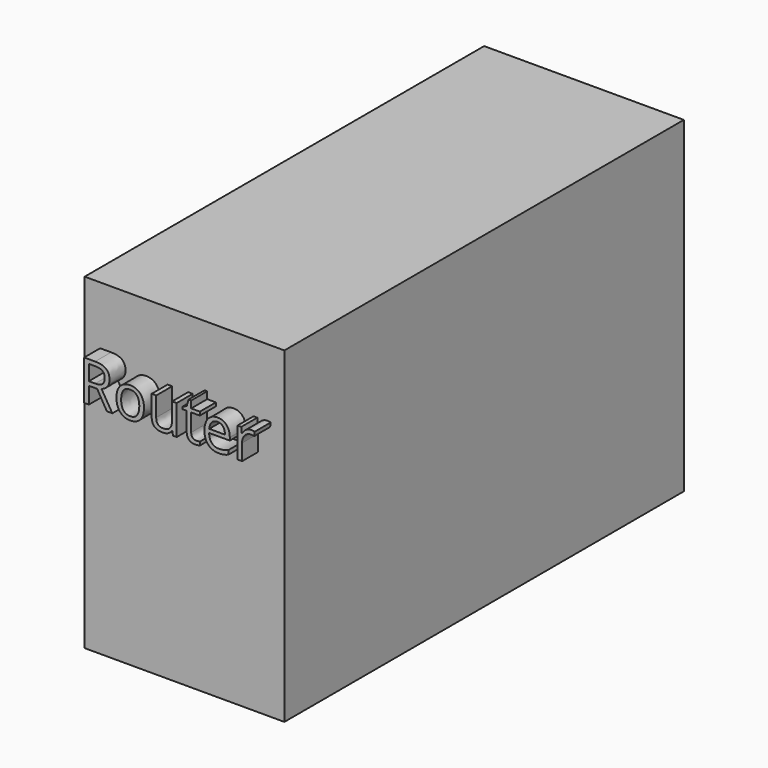
from build123d import *

# Parameters (mm, degrees)
F0_W         = 254
F0_H         = 415.925
F1_DEPTH     = 635
F2_TEXT_SIZE = 71.2392267615
F3_DEPTH     = 25.4


# Not quite as in the source:
# - Text() gives the source's letters only with a copy of the font that has no kerning and outlines rounded to 1/6400 em; it was checked with that copy


with BuildPart() as f1:
    # F0 (on Front) → F1 (new body)
    with BuildSketch(Plane.XZ):
        Rectangle(F0_W, F0_H)
    extrude(amount=F1_DEPTH)

    # F2 (on face) → F3 (join)
    with BuildSketch(Plane.XZ.offset(635)):
        with Locations((-114.3, 83.3292940016)):
            Text('Router', F2_TEXT_SIZE, font='Open Sans', text_align=(TextAlign.LEFT, TextAlign.BOTTOM))
    extrude(amount=F3_DEPTH)


solid = f1.part
